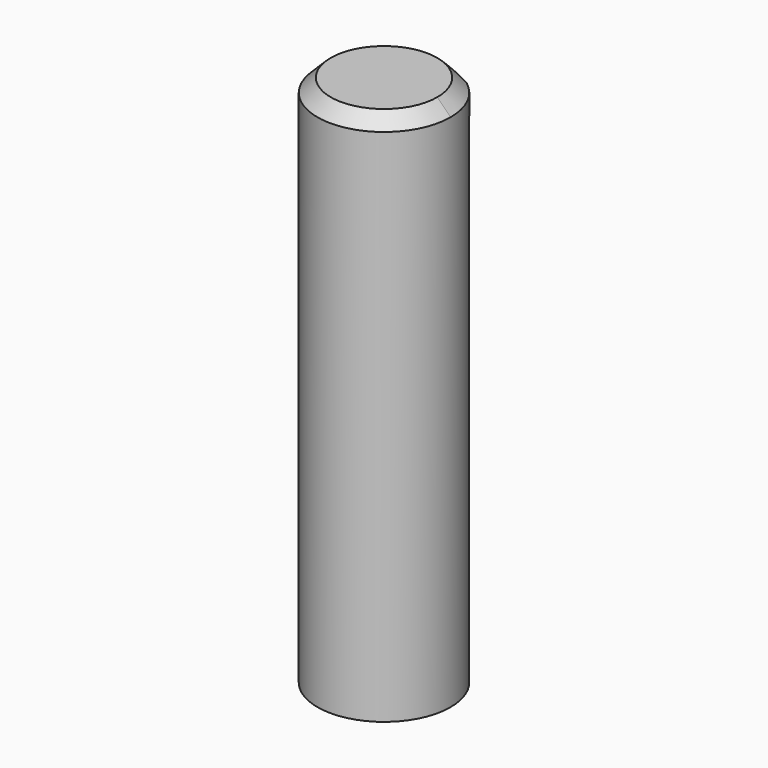
from build123d import *

# Parameters (mm, degrees)
F0_R        = 2.5
F1_DEPTH    = 20
F3_DEPTH    = 16
F4_T2_ANGLE = 304.0474034012
F4_T4_ANGLE = 123.8663608487
F5_SIZE     = 0.49999


# Not quite as in the source:
# - a fillet or chamfer that OpenCascade refuses, or shapes differently, is made with other operations: its cross-section is extruded or revolved along the edge and cut away or added
# - a fillet or chamfer is up to 0.001 mm smaller than in the source, because OpenCascade refuses the exact size


with BuildPart() as f1:
    # F0 (on Top) → F1 (new body)
    with BuildSketch(Plane.XY):
        Circle(F0_R)
    extrude(amount=F1_DEPTH)

    # F2 (on face) → F3 (cut)
    with BuildSketch(Plane.XY.offset(20)):
        with BuildLine():
            ThreePointArc((1.5, 2), (0, 2.5), (-1.5, 2))
            Line((-1.5, 2), (1.5, 2))
        make_face()
    extrude(amount=-F3_DEPTH, mode=Mode.SUBTRACT)

    # F4: chamfer of 0.5 on 1 edges, made by hand

    # F4_s1 → F4_t2 (revolve, cut)
    with BuildSketch(Plane(origin=(0, 0, 0), x_dir=(0, 0, 1), z_dir=(0.8285746432, -0.5598786125, 0))):
        with BuildLine():
            Line((19.4858578644, -2.5141421356), (20.0141421356, -1.9858578644))
            Line((20.0141421356, -1.9858578644), (20.0241421356, -1.9858578644))
            ThreePointArc((20.0241421356, -1.9858578644), (20.01, -2.2429289322), (20.01, -2.5))
            Line((20.01, -2.5), (20, -2.51))
            ThreePointArc((20, -2.51), (19.7429289322, -2.51), (19.4858578644, -2.5241421356))
            Line((19.4858578644, -2.5241421356), (19.4858578644, -2.5141421356))
        make_face()
    revolve(axis=Axis((0, 0, 20), (0, 0, 1)), revolution_arc=F4_T2_ANGLE, mode=Mode.SUBTRACT)

    # F4_s3 → F4_t4 (revolve, cut)
    with BuildSketch(Plane.XZ):
        with BuildLine():
            Line((2.5141421356, 19.4858578644), (1.9858578644, 20.0141421356))
            Line((1.9858578644, 20.0141421356), (1.9858578644, 20.0241421356))
            ThreePointArc((1.9858578644, 20.0241421356), (2.2429289322, 20.01), (2.5, 20.01))
            Line((2.5, 20.01), (2.51, 20))
            ThreePointArc((2.51, 20), (2.51, 19.7429289322), (2.5241421356, 19.4858578644))
            Line((2.5241421356, 19.4858578644), (2.5141421356, 19.4858578644))
        make_face()
    revolve(axis=Axis((0, 0, 20), (0, 0, 1)), revolution_arc=F4_T4_ANGLE, mode=Mode.SUBTRACT)

    # F5 (size 0.5 in the source; OpenCascade refuses exactly that, so slightly less here)
    f5_edges = [f1.edges().sort_by_distance(p)[0] for p in [
        (0, 2, 4),
    ]]
    chamfer(f5_edges, length=F5_SIZE)


solid = f1.part
